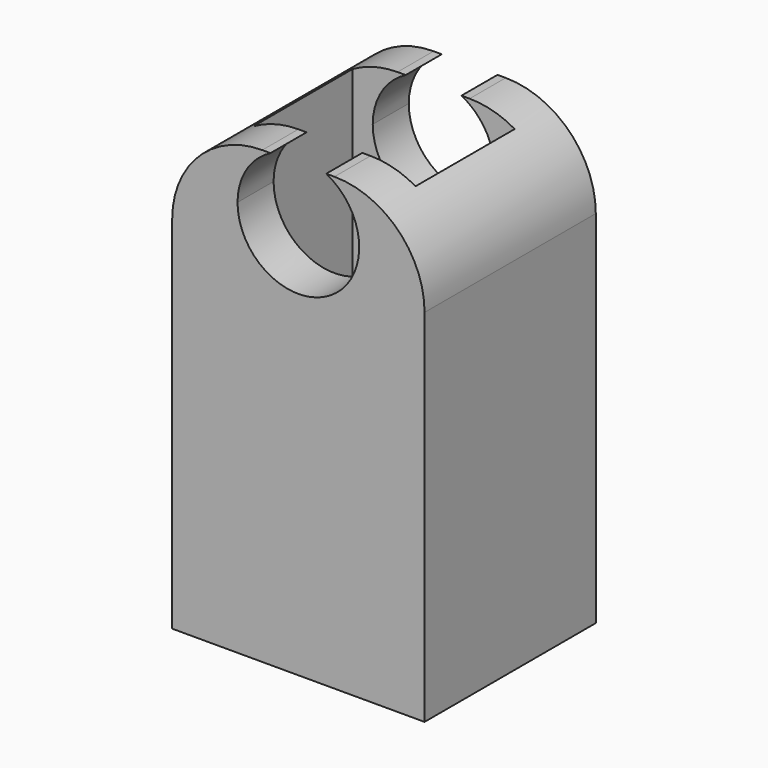
from build123d import *

# Parameters (mm, degrees)
F0_W        = 14.224
F0_H        = 12.065
F0_W_2      = 9.144
F0_H_2      = 6.985
F1_DEPTH    = 25.4
F3_DEPTH    = 8.89
F5_DEPTH    = 25.4
F6_T1_DEPTH = 37.465


# Not quite as in the source:
# - a fillet or chamfer that OpenCascade refuses, or shapes differently, is made with other operations: its cross-section is extruded or revolved along the edge and cut away or added


with BuildPart() as f1:
    # F0 (on Top) → F1 (new body)
    with BuildSketch(Plane.XY):
        Rectangle(F0_W, F0_H)
        Rectangle(F0_W_2, F0_H_2, mode=Mode.SUBTRACT)
    extrude(amount=F1_DEPTH)

    # F2 (on face) → F3 (join)
    with BuildSketch(Plane(origin=(0, -3.4925, 0), x_dir=(-1, 0, 0), z_dir=(0, 1, 0))):
        with BuildLine():
            Line((3.801523905, 13.97), (-3.801523905, 13.97))
            ThreePointArc((-3.801523905, 13.97), (-4.3751429287, 12.7571429287), (-4.572, 11.43))
            Line((-4.572, 11.43), (4.572, 11.43))
            ThreePointArc((4.572, 11.43), (4.3751429287, 12.7571429287), (3.801523905, 13.97))
        make_face()
        with BuildLine():
            Line((-3.801523905, 13.97), (-4.572, 13.97))
            Line((-4.572, 13.97), (-4.572, 11.43))
            ThreePointArc((-4.572, 11.43), (-4.3751429287, 12.7571429287), (-3.801523905, 13.97))
        make_face()
        with BuildLine():
            Line((4.572, 13.97), (3.801523905, 13.97))
            ThreePointArc((3.801523905, 13.97), (4.3751429287, 12.7571429287), (4.572, 11.43))
            Line((4.572, 11.43), (4.572, 13.97))
        make_face()
        with BuildLine():
            Line((4.572, 11.43), (-4.572, 11.43))
            ThreePointArc((-4.572, 11.43), (0, 6.858), (4.572, 11.43))
        make_face()
    extrude(amount=F3_DEPTH)

    # F4 (on face) → F5 (cut)
    with BuildSketch(Plane(origin=(0, 6.0325, 0), x_dir=(-1, 0, 0), z_dir=(0, 1, 0))):
        with BuildLine():
            ThreePointArc((-1.5709032434, 25.4), (-1.784854865, 19.424145135), (3.429, 22.352))
            ThreePointArc((3.429, 22.352), (2.927854865, 24.136854865), (1.5709032434, 25.4))
            Line((1.5709032434, 25.4), (-1.5709032434, 25.4))
        make_face()
    extrude(amount=-F5_DEPTH, mode=Mode.SUBTRACT)

    # F6: fillet of radius 5.08 on 2 edges, made by hand

    # F6_s2 → F6_t1 (cut)
    with BuildSketch(Plane.XZ.offset(-18.7325)):
        with BuildLine():
            ThreePointArc((7.112, 20.32), (5.6241024484, 23.9121024484), (2.032, 25.4))
            Line((2.032, 25.4), (7.112, 25.4))
            Line((7.112, 25.4), (7.112, 20.32))
        make_face()
        with BuildLine():
            ThreePointArc((-2.032, 25.4), (-5.6241024484, 23.9121024484), (-7.112, 20.32))
            Line((-7.112, 20.32), (-7.112, 25.4))
            Line((-7.112, 25.4), (-2.032, 25.4))
        make_face()
    extrude(amount=F6_T1_DEPTH, mode=Mode.SUBTRACT)


solid = f1.part
